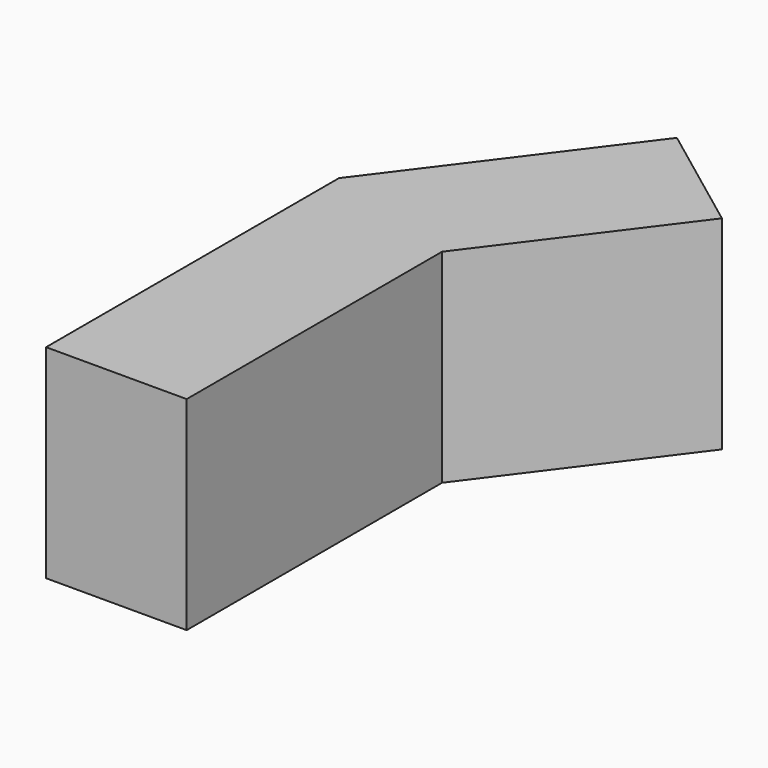
from build123d import *

# Parameters (mm, degrees)
F0_W = 40.0777868927
F0_H = 57.9875484109


with BuildPart() as f2:
    # F2: sweep along a path in F1
    with BuildLine(Plane.XY) as f2_path:
        Line((-40.0777868927, 0), (-40.0777868927, 104.355700314))
        Line((-40.0777868927, 104.355700314), (6.5287379548, 166.5153428912))
    # F0 (on Front) → F2 (sweep)
    with BuildSketch(Plane.XZ):
        with Locations((-20.0388934463, 28.9937742054)):
            Rectangle(F0_W, F0_H)
    sweep(path=f2_path.line, transition=Transition.RIGHT)


solid = f2.part
